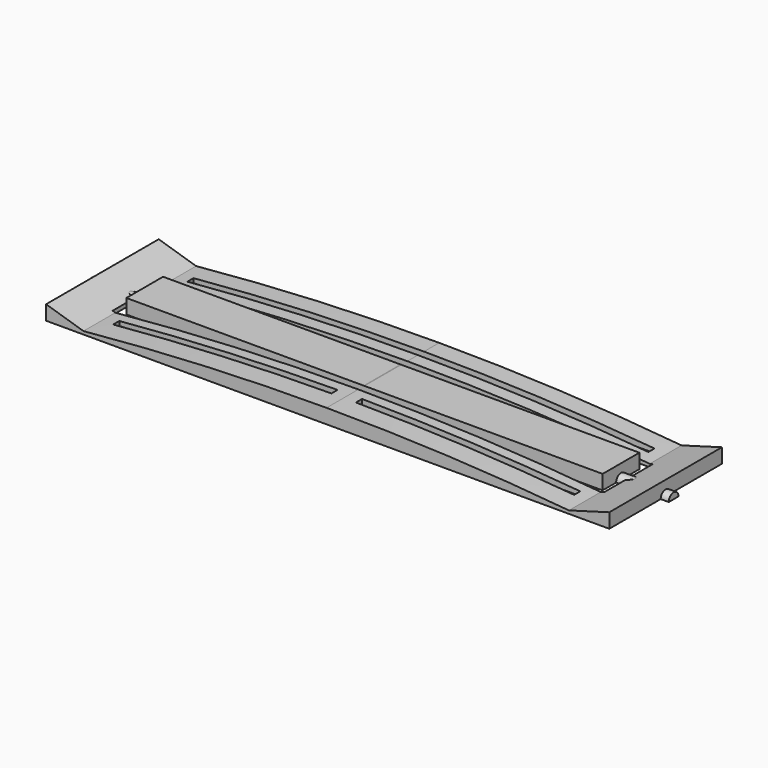
from build123d import *

# Parameters (mm, degrees)
F3_DEPTH      = 23
F3_DEPTH_BACK = 23
F2_W          = 71.3
F2_H          = 2.5
F2_W_2        = 160.6
F2_H_2        = 20
F2_W_3        = 155.6
F2_H_3        = 15
F2_W_4        = 150.6
F4_DEPTH      = 5
F7_DEPTH      = 95
F7_DEPTH_BACK = 95
F8_DEPTH      = 12
F8_DEPTH_BACK = 12
F9_DEPTH      = 4.75


# Not quite as in the source:
# - a feature names something its author has since deleted; it is built from what else it names


with BuildPart() as f3:
    # F0 (on Front) → F3 (new body, two sides)
    with BuildSketch(Plane.XZ) as f3_sk:
        with BuildLine():
            Line((0, 1.5), (0, 0))
            Line((0, 0), (1.5, 0))
            ThreePointArc((1.5, 0), (1.0606601718, 1.0606601718), (0, 1.5))
        make_face()
        with BuildLine():
            ThreePointArc((0, 1.5), (-1.0606601718, 1.0606601718), (-1.5, 0))
            Line((-1.5, 0), (0, 0))
            Line((0, 0), (0, 1.5))
        make_face()
        with BuildLine():
            Line((-91.6240630262, 0), (-79.4154876804, 0))
            Line((-79.4154876804, 0), (-1.5, 0))
            ThreePointArc((-1.5, 0), (-1.0606601718, 1.0606601718), (0, 1.5))
            Line((0, 1.5), (0, 4.75))
            ThreePointArc((0, 4.75), (-39.7521168613, 3.8147080292), (-79.4154876804, 1))
            Line((-79.4154876804, 1), (-91.6240630262, 4.75))
            Line((-91.6240630262, 4.75), (-91.6240630262, 0))
        make_face()
        with BuildLine():
            Line((0, 4.75), (0, 1.5))
            ThreePointArc((0, 1.5), (1.0606601718, 1.0606601718), (1.5, 0))
            Line((1.5, 0), (79.1845123196, 0))
            Line((79.1845123196, 0), (92.3759369738, 0))
            Line((92.3759369738, 0), (92.3759369738, 4.75))
            Line((92.3759369738, 4.75), (79.1845123196, 1))
            ThreePointArc((79.1845123196, 1), (39.6365002683, 3.8092528426), (0, 4.75))
        make_face()
    extrude(amount=F3_DEPTH)
    extrude(f3_sk.sketch, amount=-F3_DEPTH_BACK)

    # F2 (on Top) → F4 (cut)
    with BuildSketch(Plane.XY):
        with Locations((-39.65, -14.75)):
            Rectangle(F2_W, F2_H)
        with Locations((39.65, -14.75)):
            Rectangle(F2_W, F2_H)
        Rectangle(F2_W_2, F2_H_2)
        Rectangle(F2_W_3, F2_H_3, mode=Mode.SUBTRACT)
        with Locations((0, 15.5593407378)):
            Rectangle(F2_W_4, F2_H)
    extrude(amount=F4_DEPTH, mode=Mode.SUBTRACT)

    # F6 (on Right) → F7 (join, two sides)
    with BuildSketch(Plane.YZ) as f7_sk:
        with BuildLine():
            Line((-2, 0), (2, 0))
            ThreePointArc((2, 0), (0, 2), (-2, 0))
        make_face()
    extrude(amount=F7_DEPTH)
    extrude(f7_sk.sketch, amount=-F7_DEPTH_BACK)

    # F0 (on Front) → F8 (join, two sides)
    with BuildSketch(Plane.XZ) as f8_sk:
        with BuildLine():
            Line((0, 1.5), (0, 0))
            Line((0, 0), (1.5, 0))
            ThreePointArc((1.5, 0), (1.0606601718, 1.0606601718), (0, 1.5))
        make_face()
        with BuildLine():
            ThreePointArc((0, 1.5), (-1.0606601718, 1.0606601718), (-1.5, 0))
            Line((-1.5, 0), (0, 0))
            Line((0, 0), (0, 1.5))
        make_face()
    extrude(amount=F8_DEPTH)
    extrude(f8_sk.sketch, amount=-F8_DEPTH_BACK)

    # F2 (on Top) → F9 (join)
    with BuildSketch(Plane.XY):
        Rectangle(F2_W_3, F2_H_3)
    extrude(amount=F9_DEPTH)


solid = f3.part
